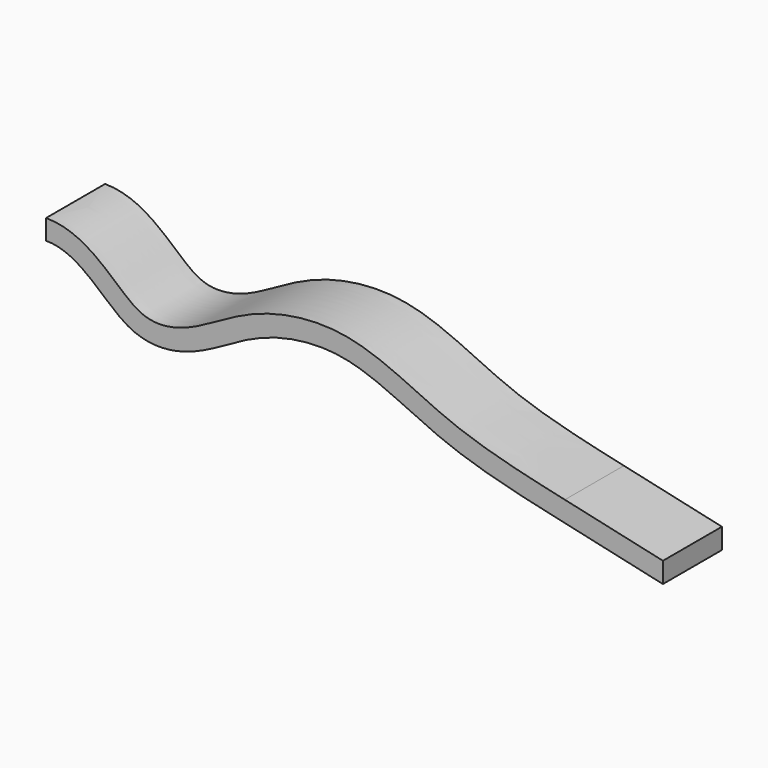
from build123d import *

# Parameters (mm, degrees)
F1_DEPTH = 23.368


# Not quite as in the source:
# - the dataset's text gives a spline's control points without its knots; the knots are read off the source's solid


with BuildPart() as f1:
    # F0 (on Front) → F1 (new body)
    with BuildSketch(Plane.XZ):
        with BuildLine():
            Line((0, 26.3227925215), (0, 19.9727928484))
            add(Edge.make_bspline(
                [(0, 19.9727928484), (11.102610788, 19.9727928484), (24.0118203246, -0.4170408168), (48.2214875777, 2.8621932512), (66.2154322806, 16.3911481519), (95.5246442906, 21.5639547504), (125.1394278308, 3.4088687327), (150.0307135552, -2.1213738435), (162.9864787767, -5.0074378938)],
                knots=[0, 0, 0, 0, 0.1723703148, 0.3141592651, 0.4616112416, 0.6244698371, 0.805160068, 1, 1, 1, 1], degree=3))
            Line((162.9864787767, -5.0074378938), (195.4344071553, -12.2356520965))
            Line((195.4344071553, -12.2356520965), (195.4344071553, -5.7300051354))
            Line((195.4344071553, -5.7300051354), (164.3671804902, 1.1906391165))
            add(Edge.make_bspline(
                [(0, 26.3227925215), (1.3930985092, 26.3227925215), (4.1068550879, 26.0659157386), (7.848996333, 25.0415413872), (11.2183253265, 23.5554560303), (14.2396111151, 21.7727388666), (16.9676597459, 19.8251977619), (19.458650937, 17.8184592472), (21.7574912325, 15.8444482238), (23.8936120995, 13.9898979295), (25.5481283987, 12.6150346283), (26.7915352586, 11.6579237344), (27.6804229187, 11.0202931775), (28.3806537167, 10.5621754408), (28.9141934427, 10.2418198595), (29.298893016, 10.0256533225), (29.6730966563, 9.8306281378), (30.1760067693, 9.5884905947), (30.8053835993, 9.3219109007), (31.5672585549, 9.0542461292), (32.595125264, 8.7631428809), (34.435142562, 8.4173137089), (37.225785803, 8.3620454215), (40.2215771883, 8.8627951842), (42.6730404965, 9.5611130291), (44.5165110348, 10.2170287339), (46.3514630911, 10.9905490092), (48.8322576024, 12.1745436809), (52.0275700179, 13.9075641285), (55.446383954, 15.8643405587), (58.3755209498, 17.4709896702), (60.6862561083, 18.6695832149), (63.1239509801, 19.832767171), (65.7129215362, 20.93051289), (68.3949109424, 21.9155268828), (72.0862734439, 23.0726290198), (76.8944825354, 24.2003666263), (81.9035808152, 24.8356921554), (85.9940241208, 25.0021832871), (89.0930275481, 24.9437168985), (91.693055933, 24.7313703034), (93.7761625359, 24.4569829862), (95.3420334816, 24.1965321097), (96.8946982873, 23.8828054107), (98.9350819627, 23.4019984243), (101.4370380597, 22.693391027), (104.3673962737, 21.7039280297), (108.1916003993, 20.2388706766), (112.8408650006, 18.2043784705), (117.377082885, 16.0669142549), (120.9679094796, 14.3860263561), (123.647300111, 13.1617536403), (126.3202169859, 11.9932805612), (128.9840255755, 10.9061272143), (131.7078333291, 9.8806229712), (135.4076068224, 8.5885233668), (140.1555637787, 7.1023954367), (146.0221971103, 5.4847305098), (154.0329342164, 3.4920794412), (160.2105412272, 2.1165842028), (164.3671804902, 1.1906391165)],
                knots=[0, 0, 0, 0, 0.015625, 0.03125, 0.046875, 0.0625, 0.078125, 0.09375, 0.109375, 0.125, 0.140625, 0.1484375, 0.15625, 0.1640625, 0.16796875, 0.171875, 0.17578125, 0.1796875, 0.1875, 0.1953125, 0.203125, 0.21875, 0.25, 0.28125, 0.296875, 0.3125, 0.328125, 0.34375, 0.375, 0.40625, 0.421875, 0.4375, 0.453125, 0.46875, 0.484375, 0.5, 0.53125, 0.5625, 0.578125, 0.59375, 0.609375, 0.6171875, 0.625, 0.6328125, 0.640625, 0.65625, 0.671875, 0.6875, 0.71875, 0.75, 0.765625, 0.78125, 0.796875, 0.8125, 0.828125, 0.84375, 0.875, 0.90625, 0.9375, 1, 1, 1, 1], degree=3))
        make_face()
    extrude(amount=F1_DEPTH)


solid = f1.part
